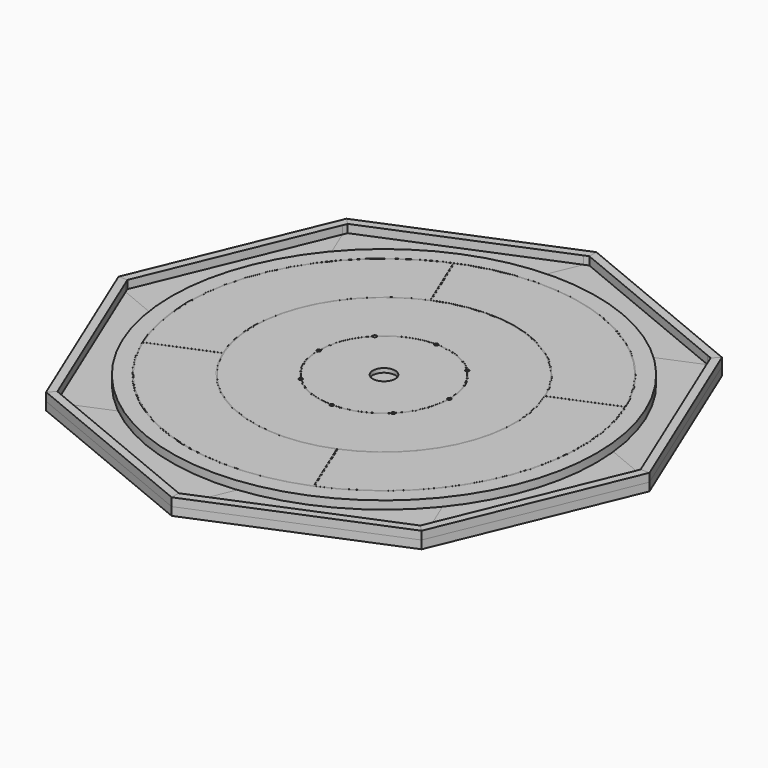
from build123d import *

# Parameters (mm, degrees)
F0_R      = 330.2
F1_DEPTH  = 12.7
F2_R      = 17.4625
F3_DEPTH  = 6.35
F4_R      = 2.794
F5_DEPTH  = 6.35
F12_DEPTH = 100.5586
F13_COUNT = 4
F15_DEPTH = 12.7
F16_COUNT = 8
F18_DEPTH = 12.7
F19_COUNT = 8


with BuildPart() as f1:
    # F0 (on Top) → F1 (new body)
    with BuildSketch(Plane.XY):
        Circle(F0_R)
    extrude(amount=F1_DEPTH)

    # F2 (on face) → F3 (cut)
    with BuildSketch(Plane.XY.offset(12.7)):
        Circle(F2_R)
    extrude(amount=-F3_DEPTH, mode=Mode.SUBTRACT)

    # F4 (on face) → F5 (cut)
    with BuildSketch(Plane.XY.offset(12.7)):
        with Locations((101.6, 0)):
            Circle(F4_R)
        with Locations((71.8420489686, 71.8420489686)):
            Circle(F4_R)
        with Locations((0, 101.6)):
            Circle(F4_R)
        with Locations((-71.8420489686, 71.8420489686)):
            Circle(F4_R)
        with Locations((-101.6, 0)):
            Circle(F4_R)
        with Locations((-71.8420489686, -71.8420489686)):
            Circle(F4_R)
        with Locations((0, -101.6)):
            Circle(F4_R)
        with Locations((71.8420489686, -71.8420489686)):
            Circle(F4_R)
    extrude(amount=-F5_DEPTH, mode=Mode.SUBTRACT)

    # F6 (on Front) → F7 (revolve, cut)
    with BuildSketch(Plane.XZ):
        with BuildLine():
            Line((-100.965, 12.7), (-102.235, 12.7))
            ThreePointArc((-102.235, 12.7), (-101.6, 12.5298522628), (-100.965, 12.7))
        make_face()
        with BuildLine():
            Line((-202.565, 12.7), (-203.835, 12.7))
            ThreePointArc((-203.835, 12.7), (-203.2, 12.5298522628), (-202.565, 12.7))
        make_face()
        with BuildLine():
            Line((-304.165, 12.7), (-305.435, 12.7))
            ThreePointArc((-305.435, 12.7), (-304.8, 12.5298522628), (-304.165, 12.7))
        make_face()
    revolve(axis=Axis((0, 0, 13.2265193388), (0, 0, 1)), mode=Mode.SUBTRACT)

    # F11 (on face) → F12 (cut)
    with BuildSketch(Plane(origin=(-78.0042774361, 188.3189845094, 0), x_dir=(0.9238795325, 0.3826834324, 0), z_dir=(0.3826834324, -0.9238795325, 0))):
        with BuildLine():
            Line((0.635, 12.7), (-0.635, 12.7))
            ThreePointArc((-0.635, 12.7), (0, 12.5298522628), (0.635, 12.7))
        make_face()
    f12 = extrude(amount=-F12_DEPTH, mode=Mode.SUBTRACT)

    # F13: F12 ×4 about axis
    f13_axis = Axis((0, 0, 12.7), (0, 0, 1))
    for i in range(1, F13_COUNT):
        add(f12.rotate(f13_axis, i * 360 / F13_COUNT), mode=Mode.SUBTRACT)


with BuildPart() as f15:
    # F14 (on face) → F15 (new body)
    with BuildSketch(Plane(origin=(0, 0, 0), x_dir=(1, 0, 0), z_dir=(0, 0, -1))):
        with BuildLine():
            Line((-256.8306230753, -207.5333010645), (-291.6469346129, -291.5873125702))
            Line((-291.6469346129, -291.5873125702), (-145.8023877311, -351.9981018868))
            Line((-145.8023877311, -351.9981018868), (-126.362069367, -305.0650216352))
            ThreePointArc((-126.362069367, -305.0650216352), (-197.7050050319, -264.470737484), (-256.8306230753, -207.5333010645))
        make_face()
        with BuildLine():
            Line((-170.8253559797, 0.1017811933), (-256.8306230753, -207.5333010645))
            ThreePointArc((-256.8306230753, -207.5333010645), (-197.7050050319, -264.470737484), (-126.362069367, -305.0650216352))
            ThreePointArc((-126.362069367, -305.0650216352), (-81.4040645489, -320.0084659426), (-34.7702792795, -328.3642302061))
            Line((-34.7702792795, -328.3642302061), (-170.8253559797, 0.1017811933))
        make_face()
        with BuildLine():
            Line((-126.362069367, -305.0650216352), (-145.8023877311, -351.9981018868))
            Line((-145.8023877311, -351.9981018868), (0.0421591507, -412.4088912034))
            Line((0.0421591507, -412.4088912034), (-34.7702792795, -328.3642302061))
            ThreePointArc((-34.7702792795, -328.3642302061), (-81.4040645489, -320.0084659426), (-126.362069367, -305.0650216352))
        make_face()
    extrude(amount=F15_DEPTH)


with BuildPart() as f16_1:
    # F16: instance of F15
    add(f15.part.rotate(Axis((0, 0, 0), (0, 0, -1)), 1 * 360 / F16_COUNT))


with BuildPart() as f16_2:
    # F16: instance of F15
    add(f15.part.rotate(Axis((0, 0, 0), (0, 0, -1)), 2 * 360 / F16_COUNT))


with BuildPart() as f16_3:
    # F16: instance of F15
    add(f15.part.rotate(Axis((0, 0, 0), (0, 0, -1)), 3 * 360 / F16_COUNT))


with BuildPart() as f16_4:
    # F16: instance of F15
    add(f15.part.rotate(Axis((0, 0, 0), (0, 0, -1)), 4 * 360 / F16_COUNT))


with BuildPart() as f16_5:
    # F16: instance of F15
    add(f15.part.rotate(Axis((0, 0, 0), (0, 0, -1)), 5 * 360 / F16_COUNT))


with BuildPart() as f16_6:
    # F16: instance of F15
    add(f15.part.rotate(Axis((0, 0, 0), (0, 0, -1)), 6 * 360 / F16_COUNT))


with BuildPart() as f16_7:
    # F16: instance of F15
    add(f15.part.rotate(Axis((0, 0, 0), (0, 0, -1)), 7 * 360 / F16_COUNT))


with BuildPart() as f18:
    # F17 (on face) → F18 (new body)
    with BuildSketch(Plane.XY):
        Polygon((-291.5873125702, 291.6469346129), (-412.4088912034, -0.0421591507), (-398.6625102597, -0.0421591507), (-284.7141220984, 275.0535849589), align=None)
        Polygon((-281.8671533881, 281.9267754308), (-291.5873125702, 291.6469346129), (-284.7141220984, 275.0535849589), align=None)
    extrude(amount=F18_DEPTH)


with BuildPart() as f19_1:
    # F19: instance of F18
    add(f18.part.rotate(Axis((0, 0, 0), (0, 0, -1)), 1 * 360 / F19_COUNT))


with BuildPart() as f19_2:
    # F19: instance of F18
    add(f18.part.rotate(Axis((0, 0, 0), (0, 0, -1)), 2 * 360 / F19_COUNT))


with BuildPart() as f19_3:
    # F19: instance of F18
    add(f18.part.rotate(Axis((0, 0, 0), (0, 0, -1)), 3 * 360 / F19_COUNT))


with BuildPart() as f19_4:
    # F19: instance of F18
    add(f18.part.rotate(Axis((0, 0, 0), (0, 0, -1)), 4 * 360 / F19_COUNT))


with BuildPart() as f19_5:
    # F19: instance of F18
    add(f18.part.rotate(Axis((0, 0, 0), (0, 0, -1)), 5 * 360 / F19_COUNT))


with BuildPart() as f19_6:
    # F19: instance of F18
    add(f18.part.rotate(Axis((0, 0, 0), (0, 0, -1)), 6 * 360 / F19_COUNT))


with BuildPart() as f19_7:
    # F19: instance of F18
    add(f18.part.rotate(Axis((0, 0, 0), (0, 0, -1)), 7 * 360 / F19_COUNT))


solid = Compound([f1.part, f15.part, f16_1.part, f16_2.part, f16_3.part, f16_4.part, f16_5.part, f16_6.part, f16_7.part, f18.part, f19_1.part, f19_2.part, f19_3.part, f19_4.part, f19_5.part, f19_6.part, f19_7.part])
